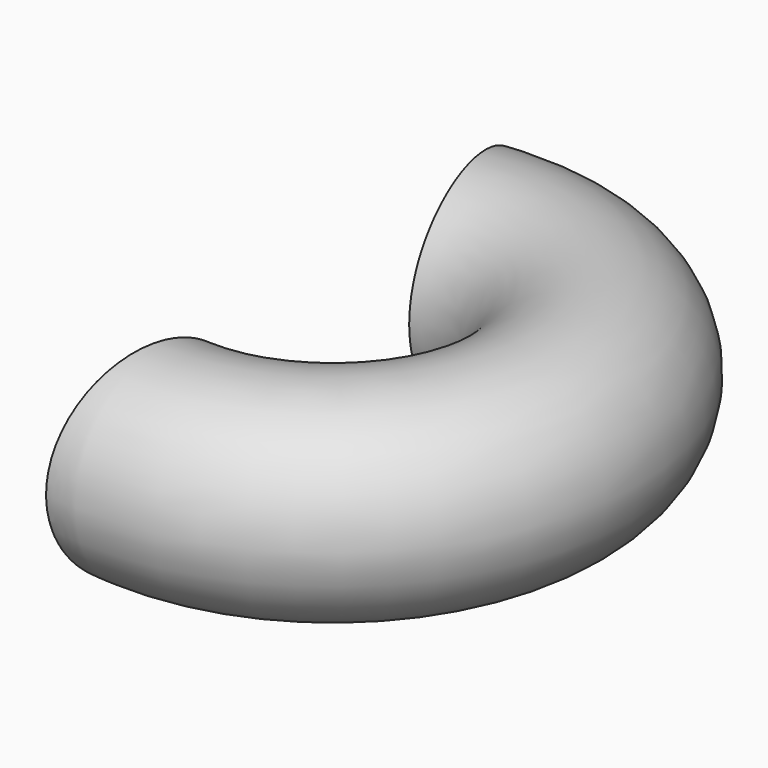
from build123d import *

# Parameters (mm, degrees)
F0_R     = 15
F3_DEPTH = 30


# Not quite as in the source:
# - a feature of the source that left no trace in its solid (it failed there, or was rolled back) is left out


with BuildPart() as f1:
    # F0 (on Front) → F1 (revolve)
    with BuildSketch(Plane.XZ):
        Circle(F0_R)
    revolve(axis=Axis((30, 0, 2.6413016021), (0, 0, -1)))


with BuildPart() as f3:
    # F2 (on Top) → F3 (new body, symmetric)
    with BuildSketch(Plane.XY):
        with BuildLine():
            add(Edge.make_bspline(
                [(0, -70), (51.9615242271, -70), (25.9807621135, 35), (0, 140), (-25.9807621135, 35), (-51.9615242271, -70), (0, -70)],
                knots=[0, 0, 0, 2.0943951024, 2.0943951024, 4.1887902048, 4.1887902048, 6.2831853072, 6.2831853072, 6.2831853072], degree=2, weights=[1, 0.5, 1, 0.5, 1, 0.5, 1]))
        make_face()
    extrude(amount=F3_DEPTH, both=True)


with BuildPart() as f1_1:
    add(f1.part)

    # F5: cut F3
    add(f3.part, mode=Mode.SUBTRACT)


solid = f1_1.part
